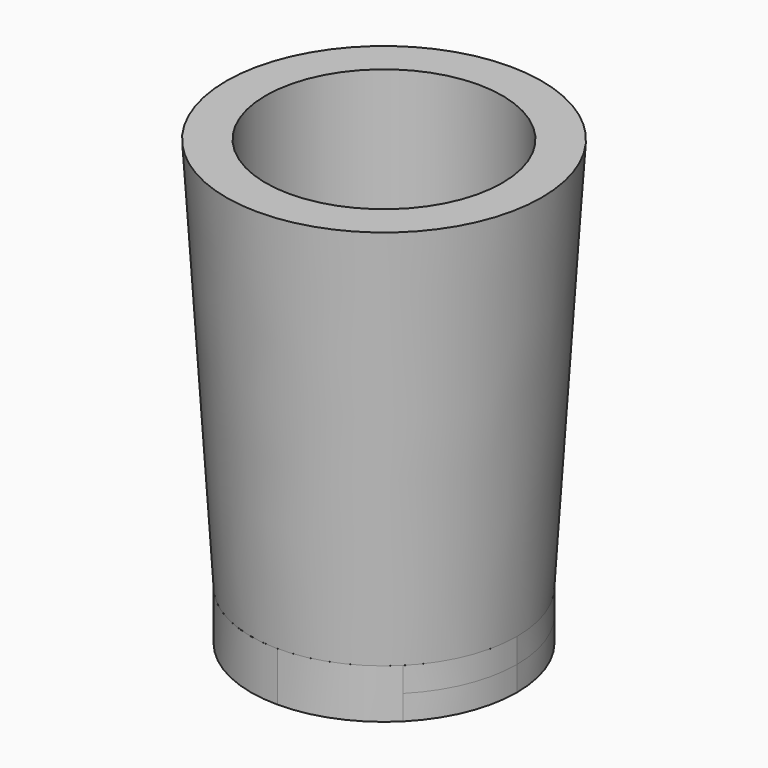
from build123d import *

# Parameters (mm, degrees)
F0_R      = 67.5
F2_R      = 80
F4_R      = 60
F5_DEPTH  = 200
F14_DEPTH = 12.5
F15_DEPTH = 12.5


# Not quite as in the source:
# - ends of sketch curves that miss each other by under 0.0002 mm in the source are joined


with BuildPart() as f3:
    # F0 (on Top) → F3 section 0
    with BuildSketch(Plane.XY):
        Circle(F0_R)
    # F2 (on offset) → F3 section 1
    with BuildSketch(Plane.XY.offset(200)):
        Circle(F2_R)
    loft()

    # F4 (on face) → F5 (cut)
    with BuildSketch(Plane.XY.offset(200)):
        Circle(F4_R)
    extrude(amount=-F5_DEPTH, mode=Mode.SUBTRACT)


with BuildPart() as f8:
    # F7 (on offset) → F8 (revolve)
    with BuildSketch(Plane.XY.offset(-12.5)):
        with BuildLine():
            ThreePointArc((48.310355393, 35.5824333316), (45.4972526643, 39.1152144312), (42.4264068712, 42.4264068712))
            Line((42.4264068712, 42.4264068712), (38.4108605979, 38.4108605979))
            ThreePointArc((38.4108605979, 38.4108605979), (41.4709466498, 35.0848828944), (44.2439582044, 31.5160369677))
            Line((44.2439582044, 31.5160369677), (48.310355393, 35.5824333316))
        make_face()
    revolve(axis=Axis((45.6196608726, 45.6196608726, -12.5), (0.7071067812, 0.7071067812, 0)))


with BuildPart() as f9:
    # F7 (on offset) → F9 (revolve)
    with BuildSketch(Plane.XY.offset(-12.5)):
        with BuildLine():
            ThreePointArc((-9, -59.3211597999), (-4.5127825124, -59.8300492562), (0, -60))
            Line((0, -60), (0, -54.32116))
            ThreePointArc((0, -54.32116), (-4.5156292812, -54.1331461855), (-9, -53.5704062309))
            Line((-9, -53.5704062309), (-9, -59.3211597999))
        make_face()
    revolve(axis=Axis((0, -9.3066766858, -12.5), (0, -1, 0)))


with BuildPart() as f9b:
    # F7 (on offset) → F9, piece 2 (revolve)
    with BuildSketch(Plane.XY.offset(-12.5)):
        with BuildLine():
            ThreePointArc((9, 59.3211597999), (4.5127825124, 59.8300492562), (0, 60))
            Line((0, 60), (0, 54.32116))
            ThreePointArc((0, 54.32116), (4.5156289866, 54.1331462101), (8.9999994169, 53.5704063289))
            Line((8.9999994169, 53.5704063289), (9, 59.3211597999))
        make_face()
    revolve(axis=Axis((0, -9.3066766858, -12.5), (0, -1, 0)))


with BuildPart() as f10:
    # F7 (on offset) → F10 (revolve)
    with BuildSketch(Plane.XY.offset(-12.5)):
        with BuildLine():
            ThreePointArc((35.582611792, -48.3102239496), (39.1152984656, -45.4971804176), (42.4264068712, -42.4264068712))
            Line((42.4264068712, -42.4264068712), (38.4108605979, -38.4108605979))
            ThreePointArc((38.4108605979, -38.4108605979), (35.0849674891, -41.4708750816), (31.5162174701, -44.2438296277))
            Line((31.5162174701, -44.2438296277), (35.582611792, -48.3102239496))
        make_face()
    revolve(axis=Axis((39.3175072968, -39.3175072968, -12.5), (0.7071067812, -0.7071067812, 0)))


with BuildPart() as f11:
    # F7 (on offset) → F11 (revolve)
    with BuildSketch(Plane.XY.offset(-12.5)):
        with BuildLine():
            ThreePointArc((-35.5824333316, 48.310355393), (-39.1152144312, 45.4972526643), (-42.4264068712, 42.4264068712))
            Line((-42.4264068712, 42.4264068712), (-38.4108605979, 38.4108605979))
            ThreePointArc((-38.4108605979, 38.4108605979), (-35.0848828944, 41.4709466498), (-31.5160369677, 44.2439582044))
            Line((-31.5160369677, 44.2439582044), (-35.5824333316, 48.310355393))
        make_face()
    revolve(axis=Axis((-40.7037734985, 40.7037734985, -12.5), (-0.7071067812, 0.7071067812, 0)))


with BuildPart() as f12:
    # F7 (on offset) → F12 (revolve)
    with BuildSketch(Plane.XY.offset(-12.5)):
        with BuildLine():
            ThreePointArc((59.3211597999, -9), (59.8300492562, -4.5127825124), (60, 0))
            Line((60, 0), (54.32116, 0))
            ThreePointArc((54.32116, 0), (54.1331462101, -4.5156289866), (53.5704063289, -8.9999994169))
            Line((53.5704063289, -8.9999994169), (59.3211597999, -9))
        make_face()
    revolve(axis=Axis((7.4657537043, 0, -12.5), (1, 0, 0)))


with BuildPart() as f12b:
    # F7 (on offset) → F12, piece 2 (revolve)
    with BuildSketch(Plane.XY.offset(-12.5)):
        with BuildLine():
            Line((-60, 0), (-54.32116, 0))
            ThreePointArc((-54.32116, 0), (-54.1331461855, 4.5156292812), (-53.5704062309, 9))
            Line((-53.5704062309, 9), (-59.3211597999, 9))
            ThreePointArc((-59.3211597999, 9), (-59.8300492562, 4.5127825124), (-60, 0))
        make_face()
    revolve(axis=Axis((7.4657537043, 0, -12.5), (1, 0, 0)))


with BuildPart() as f13:
    # F7 (on offset) → F13 (revolve)
    with BuildSketch(Plane.XY.offset(-12.5)):
        with BuildLine():
            ThreePointArc((-48.310355393, -35.5824333316), (-45.4972526643, -39.1152144312), (-42.4264068712, -42.4264068712))
            Line((-42.4264068712, -42.4264068712), (-38.4108605979, -38.4108605979))
            ThreePointArc((-38.4108605979, -38.4108605979), (-41.4709466498, -35.0848828944), (-44.2439582044, -31.5160369677))
            Line((-44.2439582044, -31.5160369677), (-48.310355393, -35.5824333316))
        make_face()
    revolve(axis=Axis((-38.4108605979, -38.4108605979, -12.5), (-0.7071067812, -0.7071067812, 0)))


with BuildPart() as f14:
    # F7 (on offset) → F14 (new body, symmetric)
    with BuildSketch(Plane.XY.offset(-12.5)):
        with BuildLine():
            ThreePointArc((0, -67.5), (25.8311316846, -62.3618684445), (47.7297077301, -47.7297077301))
            Line((47.7297077301, -47.7297077301), (42.4264068712, -42.4264068712))
            ThreePointArc((42.4264068712, -42.4264068712), (39.1152984656, -45.4971804176), (35.582611792, -48.3102239496))
            ThreePointArc((35.582611792, -48.3102239496), (18.7268064953, -57.0026904495), (0, -60))
            Line((0, -60), (0, -67.5))
        make_face()
        with BuildLine():
            ThreePointArc((-47.7297077301, -47.7297077301), (-25.8311316846, -62.3618684445), (0, -67.5))
            Line((0, -67.5), (0, -60))
            ThreePointArc((0, -60), (-4.5127825124, -59.8300492562), (-9, -59.3211597999))
            ThreePointArc((-9, -59.3211597999), (-27.0652360058, -53.5487908355), (-42.4264068712, -42.4264068712))
            Line((-42.4264068712, -42.4264068712), (-47.7297077301, -47.7297077301))
        make_face()
        with BuildLine():
            ThreePointArc((-67.5, 0), (-62.3618684445, -25.8311316846), (-47.7297077301, -47.7297077301))
            Line((-47.7297077301, -47.7297077301), (-42.4264068712, -42.4264068712))
            ThreePointArc((-42.4264068712, -42.4264068712), (-45.4972526643, -39.1152144312), (-48.310355393, -35.5824333316))
            ThreePointArc((-48.310355393, -35.5824333316), (-57.0027250383, -18.72670121), (-60, 0))
            Line((-60, 0), (-67.5, 0))
        make_face()
        with BuildLine():
            Line((-42.4264068712, 42.4264068712), (-47.7297077301, 47.7297077301))
            ThreePointArc((-47.7297077301, 47.7297077301), (-62.3618684445, 25.8311316846), (-67.5, 0))
            Line((-67.5, 0), (-60, 0))
            ThreePointArc((-60, 0), (-59.8300492562, 4.5127825124), (-59.3211597999, 9))
            ThreePointArc((-59.3211597999, 9), (-53.5487908355, 27.0652360058), (-42.4264068712, 42.4264068712))
        make_face()
        with BuildLine():
            Line((0, 60), (0, 67.5))
            ThreePointArc((0, 67.5), (-25.8311316846, 62.3618684445), (-47.7297077301, 47.7297077301))
            Line((-47.7297077301, 47.7297077301), (-42.4264068712, 42.4264068712))
            ThreePointArc((-42.4264068712, 42.4264068712), (-39.1152144312, 45.4972526643), (-35.5824333316, 48.310355393))
            ThreePointArc((-35.5824333316, 48.310355393), (-18.72670121, 57.0027250383), (0, 60))
        make_face()
        with BuildLine():
            Line((42.4264068712, 42.4264068712), (47.7297077301, 47.7297077301))
            ThreePointArc((47.7297077301, 47.7297077301), (25.8311316846, 62.3618684445), (0, 67.5))
            Line((0, 67.5), (0, 60))
            ThreePointArc((0, 60), (4.5127825124, 59.8300492562), (9, 59.3211597999))
            ThreePointArc((9, 59.3211597999), (27.0652360058, 53.5487908355), (42.4264068712, 42.4264068712))
        make_face()
        with BuildLine():
            Line((60, 0), (67.5, 0))
            ThreePointArc((67.5, 0), (62.3618684445, 25.8311316846), (47.7297077301, 47.7297077301))
            Line((47.7297077301, 47.7297077301), (42.4264068712, 42.4264068712))
            ThreePointArc((42.4264068712, 42.4264068712), (45.4972526643, 39.1152144312), (48.310355393, 35.5824333316))
            ThreePointArc((48.310355393, 35.5824333316), (57.0027250383, 18.72670121), (60, 0))
        make_face()
        with BuildLine():
            ThreePointArc((47.7297077301, -47.7297077301), (62.3618684445, -25.8311316846), (67.5, 0))
            Line((67.5, 0), (60, 0))
            ThreePointArc((60, 0), (59.8300492562, -4.5127825124), (59.3211597999, -9))
            ThreePointArc((59.3211597999, -9), (53.5487908355, -27.0652360058), (42.4264068712, -42.4264068712))
            Line((42.4264068712, -42.4264068712), (47.7297077301, -47.7297077301))
        make_face()
    extrude(amount=F14_DEPTH, both=True)


with BuildPart() as f15:
    # F7 (on offset) → F15 (new body, symmetric)
    with BuildSketch(Plane.XY.offset(-12.5)):
        with BuildLine():
            ThreePointArc((31.5162174701, -44.2438296277), (35.0849674891, -41.4708750816), (38.4108605979, -38.4108605979))
            Line((38.4108605979, -38.4108605979), (0, 0))
            Line((0, 0), (0, -54.32116))
            ThreePointArc((0, -54.32116), (16.5440665425, -51.7405284664), (31.5162174701, -44.2438296277))
        make_face()
        with BuildLine():
            Line((0, -54.32116), (0, 0))
            Line((0, 0), (-38.4108605979, -38.4108605979))
            ThreePointArc((-38.4108605979, -38.4108605979), (-24.8877556563, -48.2844492786), (-9, -53.5704062309))
            ThreePointArc((-9, -53.5704062309), (-4.5156292812, -54.1331461855), (0, -54.32116))
        make_face()
        with BuildLine():
            Line((-38.4108605979, -38.4108605979), (0, 0))
            Line((0, 0), (-54.32116, 0))
            ThreePointArc((-54.32116, 0), (-51.7405622138, -16.5439609993), (-44.2439582044, -31.5160369677))
            ThreePointArc((-44.2439582044, -31.5160369677), (-41.4709466498, -35.0848828944), (-38.4108605979, -38.4108605979))
        make_face()
        with BuildLine():
            Line((-54.32116, 0), (0, 0))
            Line((0, 0), (-38.4108605979, 38.4108605979))
            ThreePointArc((-38.4108605979, 38.4108605979), (-48.2844492786, 24.8877556563), (-53.5704062309, 9))
            ThreePointArc((-53.5704062309, 9), (-54.1331461855, 4.5156292812), (-54.32116, 0))
        make_face()
        with BuildLine():
            Line((-38.4108605979, 38.4108605979), (0, 0))
            Line((0, 0), (0, 54.32116))
            ThreePointArc((0, 54.32116), (-16.5439609993, 51.7405622138), (-31.5160369677, 44.2439582044))
            ThreePointArc((-31.5160369677, 44.2439582044), (-35.0848828944, 41.4709466498), (-38.4108605979, 38.4108605979))
        make_face()
        with BuildLine():
            Line((0, 0), (38.4108605979, 38.4108605979))
            ThreePointArc((38.4108605979, 38.4108605979), (24.8877553935, 48.284449414), (8.9999994169, 53.5704063289))
            ThreePointArc((8.9999994169, 53.5704063289), (4.5156289866, 54.1331462101), (0, 54.32116))
            Line((0, 54.32116), (0, 0))
        make_face()
        with BuildLine():
            Line((0, 0), (54.32116, 0))
            ThreePointArc((54.32116, 0), (51.7405622138, 16.5439609993), (44.2439582044, 31.5160369677))
            ThreePointArc((44.2439582044, 31.5160369677), (41.4709466498, 35.0848828944), (38.4108605979, 38.4108605979))
            Line((38.4108605979, 38.4108605979), (0, 0))
        make_face()
        with BuildLine():
            ThreePointArc((53.5704063289, -8.9999994169), (54.1331462101, -4.5156289866), (54.32116, 0))
            Line((54.32116, 0), (0, 0))
            Line((0, 0), (38.4108605979, -38.4108605979))
            ThreePointArc((38.4108605979, -38.4108605979), (48.284449414, -24.8877553935), (53.5704063289, -8.9999994169))
        make_face()
    extrude(amount=F15_DEPTH, both=True)


solid = Compound([f3.part, f8.part, f9.part, f9b.part, f10.part, f11.part, f12.part, f12b.part, f13.part, f14.part, f15.part])
